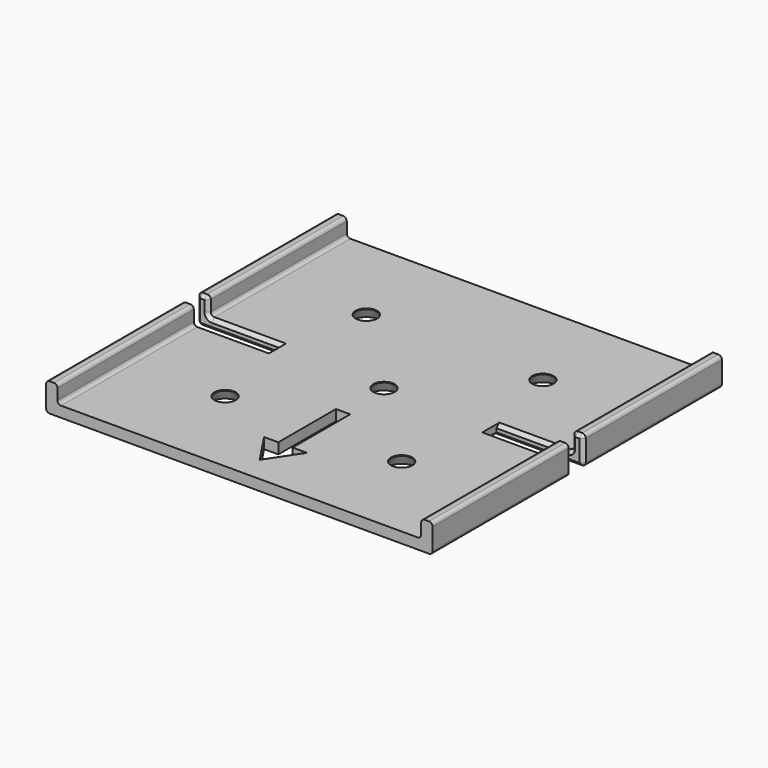
from build123d import *

# Parameters (mm, degrees)
F0_R         = 1.5
F1_DEPTH     = 1.5
F2_SIZE2     = 1.3856406461
F2_SIZE      = 0.8
F3_W         = 1.6
F3_H         = 24.3659947827
F3_H_2       = 24.4340052173
F3_H_3       = 24.4
F4_DEPTH     = 2.5
F5_R         = 0.5
F7_DEPTH     = 1.5
F8_TEXT_SIZE = 5.310416358
F9_DEPTH     = 0.5
F10_SIZE     = 0.49999


# Not quite as in the source:
# - a fillet or chamfer is up to 0.001 mm smaller than in the source, because OpenCascade refuses the exact size
# - Text() gives the source's letters only with a copy of the font that has no kerning and outlines rounded to 1/6400 em; it was checked with that copy


with BuildPart() as f1:
    # F0 (on Top) → F1 (new body)
    with BuildSketch(Plane.XY):
        Polygon((-27.15, -25.4), (27.15, -25.4), (27.15, -1), (15, -1), (15, 1), (27.15, 1), (27.15, 25.4), (-27.15, 25.4), (-27.15, 1.0340052173), (-15, 1.0340052173), (-15, -0.9659947827), (-27.15, -0.9659947827), align=None)
        with Locations((-12.4, -12.4)):
            Circle(F0_R, mode=Mode.SUBTRACT)
        with Locations((12.4, -12.4)):
            Circle(F0_R, mode=Mode.SUBTRACT)
        Circle(F0_R, mode=Mode.SUBTRACT)
        with Locations((-12.4, 12.4)):
            Circle(F0_R, mode=Mode.SUBTRACT)
        with Locations((12.4, 12.4)):
            Circle(F0_R, mode=Mode.SUBTRACT)
    extrude(amount=F1_DEPTH)

    # F2
    f2_edges = [f1.edges().sort_by_distance(p)[0] for p in [
        (-13.9, -12.4, 0),
        (10.9, -12.4, 0),
        (10.9, 12.4, 0),
        (-13.9, 12.4, 0),
        (-1.5, 0, 0),
    ]]
    f2_side = f1.faces().sort_by_distance((-21.075, -1.709576, 0))[0]
    chamfer(f2_edges, length=F2_SIZE, length2=F2_SIZE2, reference=f2_side)

    # F3 (on face) → F4 (join)
    with BuildSketch(Plane.XY.offset(1.5)):
        with Locations((-26.35, 13.2170026086)):
            Rectangle(F3_W, F3_H)
        with Locations((-26.35, -13.1829973914)):
            Rectangle(F3_W, F3_H_2)
        with Locations((26.35, -13.2)):
            Rectangle(F3_W, F3_H_3)
        with Locations((26.35, 13.2)):
            Rectangle(F3_W, F3_H_3)
    extrude(amount=F4_DEPTH)

    # F5
    f5_edges = [f1.edges().sort_by_distance(p)[0] for p in [
        (-25.55, 13.217003, 4),
        (-25.55, -13.182997, 4),
        (-27.15, 13.217003, 4),
        (-27.15, -13.182997, 4),
        (25.55, 13.2, 4),
        (25.55, -13.2, 4),
        (27.15, 13.2, 4),
        (27.15, -13.2, 4),
        (27.15, -13.2, 0),
        (27.15, 13.2, 0),
        (-27.15, -13.182997, 0),
        (-27.15, 13.217003, 0),
        (-25.55, 13.217003, 1.5),
        (-25.55, -13.182997, 1.5),
        (25.55, 13.2, 1.5),
        (25.55, -13.2, 1.5),
    ]]
    fillet(f5_edges, radius=F5_R)

    # F6 (on face) → F7 (cut)
    with BuildSketch(Plane(origin=(0, 0, 0), x_dir=(1, 0, 0), z_dir=(0, 0, -1))):
        Polygon((3, 17.3042360693), (0, 21.8301061541), (-3, 17.3042360693), (-1, 17.3042360693), (-1, 7.1805850603), (1, 7.1805850603), (1, 17.3042360693), align=None)
    extrude(amount=-F7_DEPTH, mode=Mode.SUBTRACT)

    # F8 (on face) → F9 (cut)
    with BuildSketch(Plane(origin=(0, 0, 0), x_dir=(1, 0, 0), z_dir=(0, 0, -1))):
        with Locations((-14, -22.2402960289)):
            Text('RYNO 4000', F8_TEXT_SIZE, font='Open Sans', text_align=(TextAlign.LEFT, TextAlign.BOTTOM))
    extrude(amount=-F9_DEPTH, mode=Mode.SUBTRACT)

    # F10 (size 0.5 in the source; OpenCascade refuses exactly that, so slightly less here)
    f10_edges = [f1.edges().sort_by_distance(p)[0] for p in [
        (-20.825, -0.965995, 0),
        (-15, 0.034005, 0),
        (-20.825, 1.034005, 0),
        (20.825, -1, 0),
        (15, 0, 0),
        (20.825, 1, 0),
    ]]
    chamfer(f10_edges, length=F10_SIZE)


solid = f1.part
